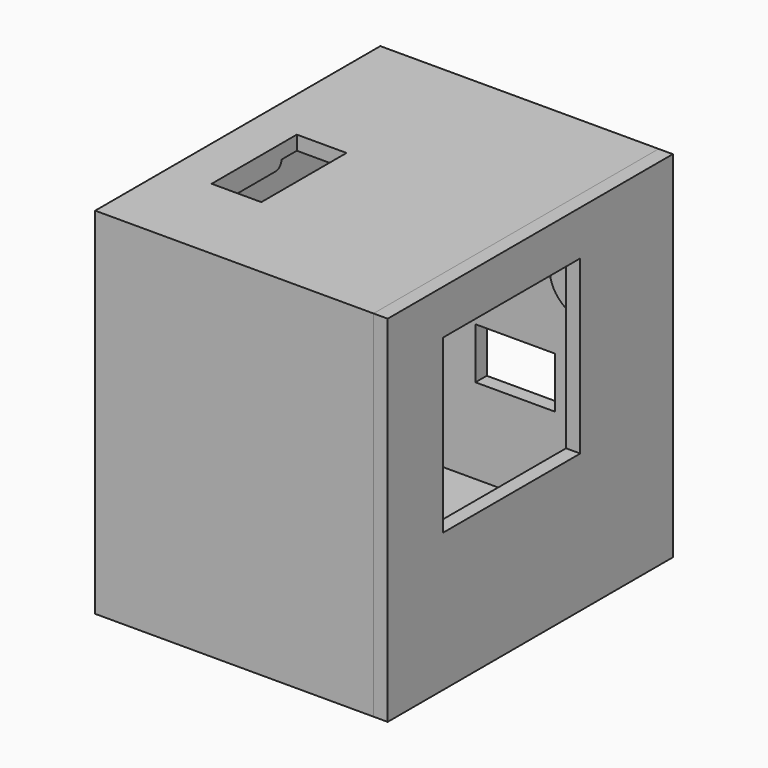
from build123d import *

# Parameters (mm, degrees)
F0_W      = 39.2
F0_H      = 50.2
F0_W_2    = 35.2
F0_H_2    = 46.2
F1_DEPTH  = 2
F2_DEPTH  = 50
F3_W      = 46.2
F3_H      = 4
F3_H_2    = 42
F4_DEPTH  = 25
F5_W      = 35.2
F5_H      = 46.2
F5_W_2    = 7
F5_H_2    = 15
F6_DEPTH  = 2
F8_DEPTH  = 1.5
F10_DEPTH = 46.2
F11_W     = 50.2
F11_H     = 50
F11_W_2   = 0.2
F11_H_2   = 1.8718592376
F11_H_3   = 18.1281407624
F11_W_3   = 2
F11_W_4   = 41.8
F12_DEPTH = 2
F13_DEPTH = 12
F14_R     = 5
F15_W     = 24.2
F15_H     = 24.2
F16_DEPTH = 5
F17_W     = 11.2
F17_H     = 7.2
F18_DEPTH = 4.5
F20_START = -10.2
F20_DEPTH = 1.5


# Not quite as in the source:
# - a feature names something its author has since deleted; it is built from what else it names


with BuildPart() as f1:
    # F0 (on Top) → F1 (new body)
    with BuildSketch(Plane.XY):
        with Locations((-3.1452118158, -2.0964890861)):
            Rectangle(F0_W, F0_H)
        with Locations((-3.1452118158, -2.0964890861)):
            Rectangle(F0_W_2, F0_H_2, mode=Mode.SUBTRACT)
        with Locations((-3.1452118158, -2.0964890861)):
            Rectangle(F0_W_2, F0_H_2)
    extrude(amount=F1_DEPTH)

    # F0 (on Top) → F2 (join)
    with BuildSketch(Plane.XY):
        with Locations((-3.1452118158, -2.0964890861)):
            Rectangle(F0_W, F0_H)
        with Locations((-3.1452118158, -2.0964890861)):
            Rectangle(F0_W_2, F0_H_2, mode=Mode.SUBTRACT)
    extrude(amount=F2_DEPTH)

    # F3 (on face) → F4 (cut)
    with BuildSketch(Plane.YZ.offset(16.4547881842)):
        with Locations((-2.0964890861, 46)):
            Rectangle(F3_W, F3_H)
        with Locations((-2.0964890861, 23)):
            Rectangle(F3_W, F3_H_2)
    extrude(amount=-F4_DEPTH, mode=Mode.SUBTRACT)

    # F5 (on face) → F6 (join)
    with BuildSketch(Plane.XY.offset(50)):
        with Locations((-3.1452118158, -2.0964890861)):
            Rectangle(F5_W, F5_H)
        with Locations((-13.2452118158, -6.6964890861)):
            Rectangle(F5_W_2, F5_H_2, mode=Mode.SUBTRACT)
    extrude(amount=-F6_DEPTH)

    # F7 (on face) → F8 (join)
    with BuildSketch(Plane.YZ.offset(-16.7452118158)):
        with BuildLine():
            ThreePointArc((-2.9464890861, 46.9503788089), (-3.688683348, 47.2578057381), (-3.9961102772, 48))
            Line((-3.9961102772, 48), (-6.6964890861, 48))
            Line((-6.6964890861, 48), (-9.396867895, 48))
            ThreePointArc((-9.396867895, 48), (-9.7042948242, 47.2578057381), (-10.4464890861, 46.9503788089))
            Line((-10.4464890861, 46.9503788089), (-2.9464890861, 46.9503788089))
        make_face()
        with BuildLine():
            ThreePointArc((-2.9464890861, 46.9503788089), (-2.2042948242, 47.2578057381), (-1.896867895, 48))
            Line((-1.896867895, 48), (-3.9961102772, 48))
            ThreePointArc((-3.9961102772, 48), (-3.688683348, 47.2578057381), (-2.9464890861, 46.9503788089))
        make_face()
        with BuildLine():
            ThreePointArc((-11.4961102772, 48), (-11.188683348, 47.2578057381), (-10.4464890861, 46.9503788089))
            ThreePointArc((-10.4464890861, 46.9503788089), (-9.7042948242, 47.2578057381), (-9.396867895, 48))
            Line((-9.396867895, 48), (-11.4961102772, 48))
        make_face()
    extrude(amount=-F8_DEPTH)

    # F9 (on face) → F10 (join, through all)
    with BuildSketch(Plane.XZ.offset(-21.0035109139)):
        Polygon((-2.6452118158, 46.1281407624), (-2.1452118158, 46.1281407624), (-1.6452118158, 46.1281407624), (-1.3952118158, 48), (-2.1452118158, 48), (-2.8952118158, 48), align=None)
    extrude(amount=F10_DEPTH)

    # F17 (on face) → F18 (cut)
    with BuildSketch(Plane.XZ.offset(-21.0035109139)):
        with Locations((-2.1452118158, 17.6)):
            Rectangle(F17_W, F17_H)
    extrude(amount=-F18_DEPTH, mode=Mode.SUBTRACT)

    # F19 (on face) → F20 (join)
    with BuildSketch(Plane.YZ.offset(16.4547881842).offset(F20_START)):
        with BuildLine():
            ThreePointArc((-11.6964890861, 48), (-11.3303725626, 47.1161165235), (-10.4464890861, 46.75))
            ThreePointArc((-10.4464890861, 46.75), (-9.5626056096, 47.1161165235), (-9.1964890861, 48))
            Line((-9.1964890861, 48), (-11.6964890861, 48))
        make_face()
        with BuildLine():
            Line((-10.4464890861, 46.75), (-2.9464890861, 46.75))
            ThreePointArc((-2.9464890861, 46.75), (-3.8303725626, 47.1161165235), (-4.1964890861, 48))
            Line((-4.1964890861, 48), (-6.6964890861, 48))
            Line((-6.6964890861, 48), (-9.1964890861, 48))
            ThreePointArc((-9.1964890861, 48), (-9.5626056096, 47.1161165235), (-10.4464890861, 46.75))
        make_face()
        with BuildLine():
            ThreePointArc((-4.1964890861, 48), (-3.8303725626, 47.1161165235), (-2.9464890861, 46.75))
            ThreePointArc((-2.9464890861, 46.75), (-2.0626056096, 47.1161165235), (-1.6964890861, 48))
            Line((-1.6964890861, 48), (-4.1964890861, 48))
        make_face()
    extrude(amount=-F20_DEPTH)


with BuildPart() as f12:
    # F11 (on face) → F12 (new body)
    with BuildSketch(Plane.YZ.offset(16.4547881842)):
        with Locations((-2.0964890861, 25)):
            Rectangle(F11_W, F11_H)
        Polygon((20.8035109139, 48), (21.0035109139, 48), (21.0035109139, 46.1281407624), (21.0035109139, 28), (21.0035109139, 2), (-25.1964890861, 2), (-25.1964890861, 28), (-25.1964890861, 46.1281407624), (-25.1964890861, 48), (-24.9964890861, 48), (-22.9964890861, 48), (18.8035109139, 48), align=None, mode=Mode.SUBTRACT)
        with Locations((20.9035109139, 47.0640703812)):
            Rectangle(F11_W_2, F11_H_2)
        with Locations((20.9035109139, 37.0640703812)):
            Rectangle(F11_W_2, F11_H_3)
        with Locations((19.8035109139, 47.0640703812)):
            Rectangle(F11_W_3, F11_H_2)
        Polygon((21.0035109139, 2), (21.0035109139, 28), (20.8035109139, 28), (18.8035109139, 28), (-22.9964890861, 28), (-24.9964890861, 28), (-25.1964890861, 28), (-25.1964890861, 2), align=None)
        with Locations((19.8035109139, 37.0640703812)):
            Rectangle(F11_W_3, F11_H_3)
        with Locations((-2.0964890861, 47.0640703812)):
            Rectangle(F11_W_4, F11_H_2)
        with Locations((-2.0964890861, 37.0640703812)):
            Rectangle(F11_W_4, F11_H_3)
        with Locations((-23.9964890861, 47.0640703812)):
            Rectangle(F11_W_3, F11_H_2)
        with Locations((-23.9964890861, 37.0640703812)):
            Rectangle(F11_W_3, F11_H_3)
        with Locations((-25.0964890861, 47.0640703812)):
            Rectangle(F11_W_2, F11_H_2)
        with Locations((-25.0964890861, 37.0640703812)):
            Rectangle(F11_W_2, F11_H_3)
    extrude(amount=F12_DEPTH)

    # F11 (on face) → F13 (join)
    with BuildSketch(Plane.YZ.offset(16.4547881842)):
        with Locations((19.8035109139, 37.0640703812)):
            Rectangle(F11_W_3, F11_H_3)
        with Locations((-23.9964890861, 37.0640703812)):
            Rectangle(F11_W_3, F11_H_3)
    extrude(amount=-F13_DEPTH)

    # F14
    f14_edges = [f12.edges().sort_by_distance(p)[0] for p in [
        (4.454788, 19.803511, 46.128141),
        (4.454788, -23.996489, 46.128141),
        (4.454788, -23.996489, 28),
        (4.454788, 19.803511, 28),
    ]]
    fillet(f14_edges, radius=F14_R)

    # F15 (on face) → F16 (cut)
    with BuildSketch(Plane.YZ.offset(18.4547881842)):
        with Locations((-5.3964890861, 31.6)):
            Rectangle(F15_W, F15_H)
    extrude(amount=-F16_DEPTH, mode=Mode.SUBTRACT)


solid = Compound([f1.part, f12.part])
